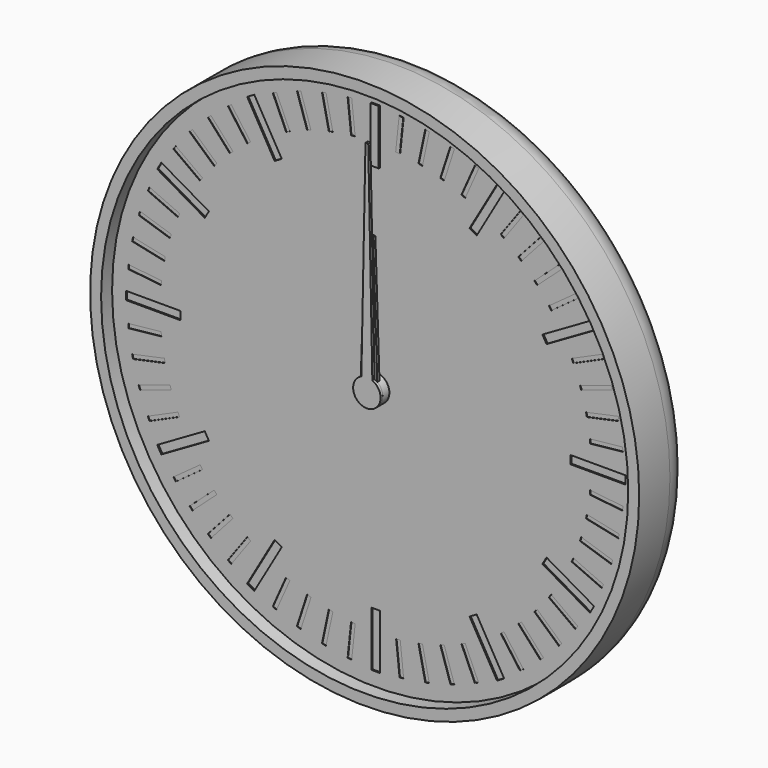
from build123d import *

# Parameters (mm, degrees)
F0_R      = 100
F1_DEPTH  = 24
F2_R      = 10
F3_T      = -4
F4_R      = 5
F4_R_2    = 3
F5_DEPTH  = 2
F6_DEPTH  = 19
F7_DEPTH  = 8
F9_DEPTH  = 4
F11_DEPTH = 4
F12_R     = 5
F12_R_2   = 3
F13_DEPTH = 2
F14_R     = 3
F15_DEPTH = 4
F17_DEPTH = 4
F18_R     = 3
F19_DEPTH = 2
F20_R     = 98
F20_R_2   = 5
F21_DEPTH = 1
F23_R     = 5
F23_R_2   = 3
F24_DEPTH = 2
F25_W     = 3
F25_H     = 20
F25_W_2   = 20
F25_H_2   = 3
F26_DEPTH = 0.5
F27_W     = 1.5
F27_H     = 12
F27_W_2   = 12
F27_H_2   = 1.5
F28_DEPTH = 0.2
F29_DEPTH = 1
F30_DEPTH = 0.4
F31_R     = 5
F31_R_2   = 3
F32_DEPTH = 5
F33_R     = 3
F34_DEPTH = 1
F36_DEPTH = 1


with BuildPart() as f1:
    # F0 (on Front) → F1 (new body)
    with BuildSketch(Plane.XZ):
        Circle(F0_R)
    extrude(amount=F1_DEPTH)

    # F2
    f2_edges = [f1.edges().sort_by_distance(p)[0] for p in [
        (-100, 0, 0),
    ]]
    fillet(f2_edges, radius=F2_R)

    # F3
    f3_openings = [f1.faces().sort_by_distance(p)[0] for p in [
        (0, -24, 0),
    ]]
    offset(amount=F3_T, openings=f3_openings)

    # F4 (on face) → F5 (join)
    with BuildSketch(Plane.XZ.offset(4)):
        Circle(F4_R)
        Circle(F4_R_2, mode=Mode.SUBTRACT)
        with Locations((40, 0)):
            Circle(F4_R)
        with Locations((40, 0)):
            Circle(F4_R_2, mode=Mode.SUBTRACT)
    extrude(amount=F5_DEPTH)


with BuildPart() as f6:
    # F6 (new): a face of the model
    f6_faces = [f1.part.faces().sort_by_distance(p)[0] for p in [
        (0, -4, 0),
    ]]
    extrude(f6_faces, amount=F6_DEPTH)

    # F8 (on face) → F9 (join)
    with BuildSketch(Plane.XZ.offset(6)):
        with BuildLine():
            ThreePointArc((9.2729637667, -1.3794085621), (9.3494561423, -0.6915886375), (9.375, 0))
            ThreePointArc((9.375, 0), (9.3494561423, 0.6915886375), (9.2729637667, 1.3794085621))
            ThreePointArc((9.2729637667, 1.3794085621), (8.9161548403, 2.8970343223), (8.3127812852, 4.3345463782))
            ThreePointArc((8.3127812852, 4.3345463782), (7.5845343223, 5.5104867402), (6.6911892658, 6.566476316))
            ThreePointArc((6.6911892658, 6.566476316), (5.5104867402, 7.5845343223), (4.1773988938, 8.3928519278))
            ThreePointArc((4.1773988938, 8.3928519278), (2.8970343223, 8.9161548403), (1.5536078905, 9.2453733036))
            ThreePointArc((1.5536078905, 9.2453733036), (0, 9.375), (-1.5536078905, 9.2453733036))
            ThreePointArc((-1.5536078905, 9.2453733036), (-2.8970343223, 8.9161548403), (-4.1773988938, 8.3928519278))
            ThreePointArc((-4.1773988938, 8.3928519278), (-5.5104867402, 7.5845343223), (-6.6911892658, 6.566476316))
            ThreePointArc((-6.6911892658, 6.566476316), (-7.5845343223, 5.5104867402), (-8.3127812852, 4.3345463782))
            ThreePointArc((-8.3127812852, 4.3345463782), (-8.9161548403, 2.8970343223), (-9.2729637667, 1.3794085621))
            ThreePointArc((-9.2729637667, 1.3794085621), (-9.375, 0), (-9.2729637667, -1.3794085621))
            ThreePointArc((-9.2729637667, -1.3794085621), (-8.9161548403, -2.8970343223), (-8.3127812852, -4.3345463782))
            ThreePointArc((-8.3127812852, -4.3345463782), (-7.5845343223, -5.5104867402), (-6.6911892658, -6.566476316))
            ThreePointArc((-6.6911892658, -6.566476316), (-5.5104867402, -7.5845343223), (-4.1773988938, -8.3928519278))
            ThreePointArc((-4.1773988938, -8.3928519278), (-2.8970343223, -8.9161548403), (-1.5536078905, -9.2453733036))
            ThreePointArc((-1.5536078905, -9.2453733036), (0, -9.375), (1.5536078905, -9.2453733036))
            ThreePointArc((1.5536078905, -9.2453733036), (2.8970343223, -8.9161548403), (4.1773988938, -8.3928519278))
            ThreePointArc((4.1773988938, -8.3928519278), (5.5104867402, -7.5845343223), (6.6911892658, -6.566476316))
            ThreePointArc((6.6911892658, -6.566476316), (7.5845343223, -5.5104867402), (8.3127812852, -4.3345463782))
            ThreePointArc((8.3127812852, -4.3345463782), (8.9161548403, -2.8970343223), (9.2729637667, -1.3794085621))
        make_face()
        with BuildLine():
            ThreePointArc((8.3127812852, 4.3345463782), (8.9161548403, 2.8970343223), (9.2729637667, 1.3794085621))
            Line((9.2729637667, 1.3794085621), (11.1823199426, 2.3946312492))
            Line((11.1823199426, 2.3946312492), (10.8182678729, 3.515068311))
            Line((10.8182678729, 3.515068311), (10.4542158031, 4.6355053728))
            Line((10.4542158031, 4.6355053728), (8.3127812852, 4.3345463782))
        make_face()
        with BuildLine():
            Line((11.1823199426, -2.3946312492), (9.2729637667, -1.3794085621))
            ThreePointArc((9.2729637667, -1.3794085621), (8.9161548403, -2.8970343223), (8.3127812852, -4.3345463782))
            Line((8.3127812852, -4.3345463782), (10.4542158031, -4.6355053728))
            Line((10.4542158031, -4.6355053728), (10.8182678729, -3.515068311))
            Line((10.8182678729, -3.515068311), (11.1823199426, -2.3946312492))
        make_face()
        with BuildLine():
            ThreePointArc((4.1773988938, 8.3928519278), (5.5104867402, 7.5845343223), (6.6911892658, 6.566476316))
            Line((6.6911892658, 6.566476316), (7.6391579371, 8.5101001246))
            Line((7.6391579371, 8.5101001246), (6.6860572448, 9.202568311))
            Line((6.6860572448, 9.202568311), (5.7329565525, 9.8950364974))
            Line((5.7329565525, 9.8950364974), (4.1773988938, 8.3928519278))
        make_face()
        with BuildLine():
            Line((7.6391579371, -8.5101001246), (6.6911892658, -6.566476316))
            ThreePointArc((6.6911892658, -6.566476316), (5.5104867402, -7.5845343223), (4.1773988938, -8.3928519278))
            Line((4.1773988938, -8.3928519278), (5.7329565525, -9.8950364974))
            Line((5.7329565525, -9.8950364974), (6.6860572448, -9.202568311))
            Line((6.6860572448, -9.202568311), (7.6391579371, -8.5101001246))
        make_face()
        with BuildLine():
            ThreePointArc((-1.5536078905, 9.2453733036), (0, 9.375), (1.5536078905, 9.2453733036))
            Line((1.5536078905, 9.2453733036), (1.1780972451, 11.375))
            Line((1.1780972451, 11.375), (0, 11.375))
            Line((0, 11.375), (-1.1780972451, 11.375))
            Line((-1.1780972451, 11.375), (-1.5536078905, 9.2453733036))
        make_face()
        with BuildLine():
            Line((1.1780972451, -11.375), (1.5536078905, -9.2453733036))
            ThreePointArc((1.5536078905, -9.2453733036), (0, -9.375), (-1.5536078905, -9.2453733036))
            Line((-1.5536078905, -9.2453733036), (-1.1780972451, -11.375))
            Line((-1.1780972451, -11.375), (0, -11.375))
            Line((0, -11.375), (1.1780972451, -11.375))
        make_face()
        with BuildLine():
            ThreePointArc((-6.6911892658, 6.566476316), (-5.5104867402, 7.5845343223), (-4.1773988938, 8.3928519278))
            Line((-4.1773988938, 8.3928519278), (-5.7329565525, 9.8950364974))
            Line((-5.7329565525, 9.8950364974), (-6.6860572448, 9.202568311))
            Line((-6.6860572448, 9.202568311), (-7.6391579371, 8.5101001246))
            Line((-7.6391579371, 8.5101001246), (-6.6911892658, 6.566476316))
        make_face()
        with BuildLine():
            Line((-5.7329565525, -9.8950364974), (-4.1773988938, -8.3928519278))
            ThreePointArc((-4.1773988938, -8.3928519278), (-5.5104867402, -7.5845343223), (-6.6911892658, -6.566476316))
            Line((-6.6911892658, -6.566476316), (-7.6391579371, -8.5101001246))
            Line((-7.6391579371, -8.5101001246), (-6.6860572448, -9.202568311))
            Line((-6.6860572448, -9.202568311), (-5.7329565525, -9.8950364974))
        make_face()
        with BuildLine():
            ThreePointArc((-9.2729637667, 1.3794085621), (-8.9161548403, 2.8970343223), (-8.3127812852, 4.3345463782))
            Line((-8.3127812852, 4.3345463782), (-10.4542158031, 4.6355053728))
            Line((-10.4542158031, 4.6355053728), (-10.8182678729, 3.515068311))
            Line((-10.8182678729, 3.515068311), (-11.1823199426, 2.3946312492))
            Line((-11.1823199426, 2.3946312492), (-9.2729637667, 1.3794085621))
        make_face()
        with BuildLine():
            Line((-10.4542158031, -4.6355053728), (-8.3127812852, -4.3345463782))
            ThreePointArc((-8.3127812852, -4.3345463782), (-8.9161548403, -2.8970343223), (-9.2729637667, -1.3794085621))
            Line((-9.2729637667, -1.3794085621), (-11.1823199426, -2.3946312492))
            Line((-11.1823199426, -2.3946312492), (-10.8182678729, -3.515068311))
            Line((-10.8182678729, -3.515068311), (-10.4542158031, -4.6355053728))
        make_face()
    extrude(amount=F9_DEPTH)

    # F35 (on face) → F36 (join)
    with BuildSketch(Plane.XZ.offset(23)):
        with BuildLine():
            ThreePointArc((-2, 4.582575695), (-2.7386127875, -4.1833001327), (5, 0))
            ThreePointArc((5, 0), (4.1833001327, 2.7386127875), (2, 4.582575695))
            ThreePointArc((2, 4.582575695), (0, 5), (-2, 4.582575695))
        make_face()
        with BuildLine():
            ThreePointArc((-2, 4.582575695), (0, 5), (2, 4.582575695))
            Line((2, 4.582575695), (0.5, 80))
            Line((0.5, 80), (0, 80))
            Line((0, 80), (-0.5, 80))
            Line((-0.5, 80), (-2, 4.582575695))
        make_face()
    extrude(amount=-F36_DEPTH)


with BuildPart() as f7:
    # F7 (new): a face of the model
    f7_faces = [f1.part.faces().sort_by_distance(p)[0] for p in [
        (40, -4, 0),
    ]]
    extrude(f7_faces, amount=F7_DEPTH)

    # F10 (on face) → F11 (join)
    with BuildSketch(Plane.XZ.offset(6)):
        with BuildLine():
            ThreePointArc((68.0829066802, -1.5381733945), (68.1144747006, -0.7693746225), (68.125, 0))
            ThreePointArc((68.125, 0), (68.1144747006, 0.7693746225), (68.0829066802, 1.5381733945))
            ThreePointArc((68.0829066802, 1.5381733945), (67.9709283072, 2.9398630294), (67.7890320221, 4.3342039956))
            ThreePointArc((67.7890320221, 4.3342039956), (67.5104012706, 5.8475163042), (67.1494235596, 7.3433252263))
            ThreePointArc((67.1494235596, 7.3433252263), (66.7484645208, 8.6911029668), (66.280643318, 10.0171558733))
            ThreePointArc((66.280643318, 10.0171558733), (65.6934659962, 11.4394680865), (65.0293803521, 12.8275385085))
            ThreePointArc((65.0293803521, 12.8275385085), (64.3569644814, 14.0625), (63.6236643925, 15.2623099717))
            ThreePointArc((63.6236643925, 15.2623099717), (62.7536029668, 16.5314602207), (61.815433119, 17.7511268046))
            ThreePointArc((61.815433119, 17.7511268046), (60.9009482166, 18.8192983038), (59.934217974, 19.8404278876))
            ThreePointArc((59.934217974, 19.8404278876), (58.8192983038, 20.9009482166), (57.6480467764, 21.8989056799))
            ThreePointArc((57.6480467764, 21.8989056799), (56.5314602207, 22.7536029668), (55.3735505752, 23.5514238999))
            ThreePointArc((55.3735505752, 23.5514238999), (54.0625, 24.3569644814), (52.709356105, 25.0895972944))
            ThreePointArc((52.709356105, 25.0895972944), (51.4394680865, 25.6934659962), (50.1409852457, 26.2331096755))
            ThreePointArc((50.1409852457, 26.2331096755), (48.6911029668, 26.7484645208), (47.2152055856, 27.1837531139))
            ThreePointArc((47.2152055856, 27.1837531139), (45.8475163042, 27.5104012706), (44.4652101991, 27.7682826779))
            ThreePointArc((44.4652101991, 27.7682826779), (42.9398630294, 27.9709283072), (41.4057159597, 28.0898484802))
            ThreePointArc((41.4057159597, 28.0898484802), (40, 28.125), (38.5942840403, 28.0898484802))
            ThreePointArc((38.5942840403, 28.0898484802), (37.0601369706, 27.9709283072), (35.5347898009, 27.7682826779))
            ThreePointArc((35.5347898009, 27.7682826779), (34.1524836958, 27.5104012706), (32.7847944144, 27.1837531139))
            ThreePointArc((32.7847944144, 27.1837531139), (31.3088970332, 26.7484645208), (29.8590147543, 26.2331096755))
            ThreePointArc((29.8590147543, 26.2331096755), (28.5605319135, 25.6934659962), (27.290643895, 25.0895972944))
            ThreePointArc((27.290643895, 25.0895972944), (25.9375, 24.3569644814), (24.6264494248, 23.5514238999))
            ThreePointArc((24.6264494248, 23.5514238999), (23.4685397793, 22.7536029668), (22.3519532236, 21.8989056799))
            ThreePointArc((22.3519532236, 21.8989056799), (21.1807016962, 20.9009482166), (20.065782026, 19.8404278876))
            ThreePointArc((20.065782026, 19.8404278876), (19.0990517834, 18.8192983038), (18.184566881, 17.7511268046))
            ThreePointArc((18.184566881, 17.7511268046), (17.2463970332, 16.5314602207), (16.3763356075, 15.2623099717))
            ThreePointArc((16.3763356075, 15.2623099717), (15.6430355186, 14.0625), (14.9706196479, 12.8275385085))
            ThreePointArc((14.9706196479, 12.8275385085), (14.3065340038, 11.4394680865), (13.719356682, 10.0171558733))
            ThreePointArc((13.719356682, 10.0171558733), (13.2515354792, 8.6911029668), (12.8505764404, 7.3433252263))
            ThreePointArc((12.8505764404, 7.3433252263), (12.4895987294, 5.8475163042), (12.2109679779, 4.3342039956))
            ThreePointArc((12.2109679779, 4.3342039956), (12.0290716928, 2.9398630294), (11.9170933198, 1.5381733945))
            ThreePointArc((11.9170933198, 1.5381733945), (11.875, 0), (11.9170933198, -1.5381733945))
            ThreePointArc((11.9170933198, -1.5381733945), (12.0290716928, -2.9398630294), (12.2109679779, -4.3342039956))
            ThreePointArc((12.2109679779, -4.3342039956), (12.4895987294, -5.8475163042), (12.8505764404, -7.3433252263))
            ThreePointArc((12.8505764404, -7.3433252263), (13.2515354792, -8.6911029668), (13.719356682, -10.0171558733))
            ThreePointArc((13.719356682, -10.0171558733), (14.3065340038, -11.4394680865), (14.9706196479, -12.8275385085))
            ThreePointArc((14.9706196479, -12.8275385085), (15.6430355186, -14.0625), (16.3763356075, -15.2623099717))
            ThreePointArc((16.3763356075, -15.2623099717), (17.2463970332, -16.5314602207), (18.184566881, -17.7511268046))
            ThreePointArc((18.184566881, -17.7511268046), (19.0990517834, -18.8192983038), (20.065782026, -19.8404278876))
            ThreePointArc((20.065782026, -19.8404278876), (21.1807016962, -20.9009482166), (22.3519532236, -21.8989056799))
            ThreePointArc((22.3519532236, -21.8989056799), (23.4685397793, -22.7536029668), (24.6264494248, -23.5514238999))
            ThreePointArc((24.6264494248, -23.5514238999), (25.9375, -24.3569644814), (27.290643895, -25.0895972944))
            ThreePointArc((27.290643895, -25.0895972944), (28.5605319135, -25.6934659962), (29.8590147543, -26.2331096755))
            ThreePointArc((29.8590147543, -26.2331096755), (31.3088970332, -26.7484645208), (32.7847944144, -27.1837531139))
            ThreePointArc((32.7847944144, -27.1837531139), (34.1524836958, -27.5104012706), (35.5347898009, -27.7682826779))
            ThreePointArc((35.5347898009, -27.7682826779), (37.0601369706, -27.9709283072), (38.5942840403, -28.0898484802))
            ThreePointArc((38.5942840403, -28.0898484802), (40, -28.125), (41.4057159597, -28.0898484802))
            ThreePointArc((41.4057159597, -28.0898484802), (42.9398630294, -27.9709283072), (44.4652101991, -27.7682826779))
            ThreePointArc((44.4652101991, -27.7682826779), (45.8475163042, -27.5104012706), (47.2152055856, -27.1837531139))
            ThreePointArc((47.2152055856, -27.1837531139), (48.6911029668, -26.7484645208), (50.1409852457, -26.2331096755))
            ThreePointArc((50.1409852457, -26.2331096755), (51.4394680865, -25.6934659962), (52.709356105, -25.0895972944))
            ThreePointArc((52.709356105, -25.0895972944), (54.0625, -24.3569644814), (55.3735505752, -23.5514238999))
            ThreePointArc((55.3735505752, -23.5514238999), (56.5314602207, -22.7536029668), (57.6480467764, -21.8989056799))
            ThreePointArc((57.6480467764, -21.8989056799), (58.8192983038, -20.9009482166), (59.934217974, -19.8404278876))
            ThreePointArc((59.934217974, -19.8404278876), (60.9009482166, -18.8192983038), (61.815433119, -17.7511268046))
            ThreePointArc((61.815433119, -17.7511268046), (62.7536029668, -16.5314602207), (63.6236643925, -15.2623099717))
            ThreePointArc((63.6236643925, -15.2623099717), (64.3569644814, -14.0625), (65.0293803521, -12.8275385085))
            ThreePointArc((65.0293803521, -12.8275385085), (65.6934659962, -11.4394680865), (66.280643318, -10.0171558733))
            ThreePointArc((66.280643318, -10.0171558733), (66.7484645208, -8.6911029668), (67.1494235596, -7.3433252263))
            ThreePointArc((67.1494235596, -7.3433252263), (67.5104012706, -5.8475163042), (67.7890320221, -4.3342039956))
            ThreePointArc((67.7890320221, -4.3342039956), (67.9709283072, -2.9398630294), (68.0829066802, -1.5381733945))
        make_face()
        with BuildLine():
            ThreePointArc((68.0829066802, 1.5381733945), (68.1144747006, 0.7693746225), (68.125, 0))
            ThreePointArc((68.125, 0), (68.1144747006, -0.7693746225), (68.0829066802, -1.5381733945))
            Line((68.0829066802, -1.5381733945), (70.125, -1.1780972451))
            Line((70.125, -1.1780972451), (70.125, 0))
            Line((70.125, 0), (70.125, 1.1780972451))
            Line((70.125, 1.1780972451), (68.0829066802, 1.5381733945))
        make_face()
        with BuildLine():
            ThreePointArc((67.1494235596, 7.3433252263), (67.5104012706, 5.8475163042), (67.7890320221, 4.3342039956))
            Line((67.7890320221, 4.3342039956), (69.7116366623, 5.1109866922))
            Line((69.7116366623, 5.1109866922), (69.4666964721, 6.2633396859))
            Line((69.4666964721, 6.2633396859), (69.2217562819, 7.4156926796))
            Line((69.2217562819, 7.4156926796), (67.1494235596, 7.3433252263))
        make_face()
        with BuildLine():
            Line((69.7116366623, -5.1109866922), (67.7890320221, -4.3342039956))
            ThreePointArc((67.7890320221, -4.3342039956), (67.5104012706, -5.8475163042), (67.1494235596, -7.3433252263))
            Line((67.1494235596, -7.3433252263), (69.2217562819, -7.4156926796))
            Line((69.2217562819, -7.4156926796), (69.4666964721, -6.2633396859))
            Line((69.4666964721, -6.2633396859), (69.7116366623, -5.1109866922))
        make_face()
        with BuildLine():
            ThreePointArc((65.0293803521, 12.8275385085), (65.6934659962, 11.4394680865), (66.280643318, 10.0171558733))
            Line((66.280643318, 10.0171558733), (67.9997322302, 11.1766959857))
            Line((67.9997322302, 11.1766959857), (67.5205569115, 12.2529413727))
            Line((67.5205569115, 12.2529413727), (67.0413815928, 13.3291867596))
            Line((67.0413815928, 13.3291867596), (65.0293803521, 12.8275385085))
        make_face()
        with BuildLine():
            Line((67.9997322302, -11.1766959857), (66.280643318, -10.0171558733))
            ThreePointArc((66.280643318, -10.0171558733), (65.6934659962, -11.4394680865), (65.0293803521, -12.8275385085))
            Line((65.0293803521, -12.8275385085), (67.0413815928, -13.3291867596))
            Line((67.0413815928, -13.3291867596), (67.5205569115, -12.2529413727))
            Line((67.5205569115, -12.2529413727), (67.9997322302, -11.1766959857))
        make_face()
        with BuildLine():
            ThreePointArc((61.815433119, 17.7511268046), (62.7536029668, 16.5314602207), (63.6236643925, 15.2623099717))
            Line((63.6236643925, 15.2623099717), (65.064105142, 16.753930033))
            Line((65.064105142, 16.753930033), (64.3716369555, 17.7070307253))
            Line((64.3716369555, 17.7070307253), (63.6791687691, 18.6601314176))
            Line((63.6791687691, 18.6601314176), (61.815433119, 17.7511268046))
        make_face()
        with BuildLine():
            Line((65.064105142, -16.753930033), (63.6236643925, -15.2623099717))
            ThreePointArc((63.6236643925, -15.2623099717), (62.7536029668, -16.5314602207), (61.815433119, -17.7511268046))
            Line((61.815433119, -17.7511268046), (63.6791687691, -18.6601314176))
            Line((63.6791687691, -18.6601314176), (64.3716369555, -17.7070307253))
            Line((64.3716369555, -17.7070307253), (65.064105142, -16.753930033))
        make_face()
        with BuildLine():
            ThreePointArc((57.6480467764, 21.8989056799), (58.8192983038, 20.9009482166), (59.934217974, 19.8404278876))
            Line((59.934217974, 19.8404278876), (61.0330563882, 21.5989369435))
            Line((61.0330563882, 21.5989369435), (60.1575595166, 22.3872378675))
            Line((60.1575595166, 22.3872378675), (59.282062645, 23.1755387915))
            Line((59.282062645, 23.1755387915), (57.6480467764, 21.8989056799))
        make_face()
        with BuildLine():
            Line((61.0330563882, -21.5989369435), (59.934217974, -19.8404278876))
            ThreePointArc((59.934217974, -19.8404278876), (58.8192983038, -20.9009482166), (57.6480467764, -21.8989056799))
            Line((57.6480467764, -21.8989056799), (59.282062645, -23.1755387915))
            Line((59.282062645, -23.1755387915), (60.1575595166, -22.3872378675))
            Line((60.1575595166, -22.3872378675), (61.0330563882, -21.5989369435))
        make_face()
        with BuildLine():
            ThreePointArc((52.709356105, 25.0895972944), (54.0625, 24.3569644814), (55.3735505752, 23.5514238999))
            Line((55.3735505752, 23.5514238999), (56.0827621424, 25.4999666665))
            Line((56.0827621424, 25.4999666665), (55.0625, 26.089015289))
            Line((55.0625, 26.089015289), (54.0422378576, 26.6780639116))
            Line((54.0422378576, 26.6780639116), (52.709356105, 25.0895972944))
        make_face()
        with BuildLine():
            Line((56.0827621424, -25.4999666665), (55.3735505752, -23.5514238999))
            ThreePointArc((55.3735505752, -23.5514238999), (54.0625, -24.3569644814), (52.709356105, -25.0895972944))
            Line((52.709356105, -25.0895972944), (54.0422378576, -26.6780639116))
            Line((54.0422378576, -26.6780639116), (55.0625, -26.089015289))
            Line((55.0625, -26.089015289), (56.0827621424, -25.4999666665))
        make_face()
        with BuildLine():
            ThreePointArc((47.2152055856, 27.1837531139), (48.6911029668, 26.7484645208), (50.1409852457, 26.2331096755))
            Line((50.1409852457, 26.2331096755), (50.4295740173, 28.2865254836))
            Line((50.4295740173, 28.2865254836), (49.3091369555, 28.6505775534))
            Line((49.3091369555, 28.6505775534), (48.1886998938, 29.0146296232))
            Line((48.1886998938, 29.0146296232), (47.2152055856, 27.1837531139))
        make_face()
        with BuildLine():
            Line((50.4295740173, -28.2865254836), (50.1409852457, -26.2331096755))
            ThreePointArc((50.1409852457, -26.2331096755), (48.6911029668, -26.7484645208), (47.2152055856, -27.1837531139))
            Line((47.2152055856, -27.1837531139), (48.1886998938, -29.0146296232))
            Line((48.1886998938, -29.0146296232), (49.3091369555, -28.6505775534))
            Line((49.3091369555, -28.6505775534), (50.4295740173, -28.2865254836))
        make_face()
        with BuildLine():
            ThreePointArc((41.4057159597, 28.0898484802), (42.9398630294, 27.9709283072), (44.4652101991, 27.7682826779))
            Line((44.4652101991, 27.7682826779), (44.3205634611, 29.8368274034))
            Line((44.3205634611, 29.8368274034), (43.1489199559, 29.959972098))
            Line((43.1489199559, 29.959972098), (41.9772764508, 30.0831167926))
            Line((41.9772764508, 30.0831167926), (41.4057159597, 28.0898484802))
        make_face()
        with BuildLine():
            Line((44.3205634611, -29.8368274034), (44.4652101991, -27.7682826779))
            ThreePointArc((44.4652101991, -27.7682826779), (42.9398630294, -27.9709283072), (41.4057159597, -28.0898484802))
            Line((41.4057159597, -28.0898484802), (41.9772764508, -30.0831167926))
            Line((41.9772764508, -30.0831167926), (43.1489199559, -29.959972098))
            Line((43.1489199559, -29.959972098), (44.3205634611, -29.8368274034))
        make_face()
        with BuildLine():
            ThreePointArc((35.5347898009, 27.7682826779), (37.0601369706, 27.9709283072), (38.5942840403, 28.0898484802))
            Line((38.5942840403, 28.0898484802), (38.0227235492, 30.0831167926))
            Line((38.0227235492, 30.0831167926), (36.8510800441, 29.959972098))
            Line((36.8510800441, 29.959972098), (35.6794365389, 29.8368274034))
            Line((35.6794365389, 29.8368274034), (35.5347898009, 27.7682826779))
        make_face()
        with BuildLine():
            Line((38.0227235492, -30.0831167926), (38.5942840403, -28.0898484802))
            ThreePointArc((38.5942840403, -28.0898484802), (37.0601369706, -27.9709283072), (35.5347898009, -27.7682826779))
            Line((35.5347898009, -27.7682826779), (35.6794365389, -29.8368274034))
            Line((35.6794365389, -29.8368274034), (36.8510800441, -29.959972098))
            Line((36.8510800441, -29.959972098), (38.0227235492, -30.0831167926))
        make_face()
        with BuildLine():
            ThreePointArc((29.8590147543, 26.2331096755), (31.3088970332, 26.7484645208), (32.7847944144, 27.1837531139))
            Line((32.7847944144, 27.1837531139), (31.8113001062, 29.0146296232))
            Line((31.8113001062, 29.0146296232), (30.6908630445, 28.6505775534))
            Line((30.6908630445, 28.6505775534), (29.5704259827, 28.2865254836))
            Line((29.5704259827, 28.2865254836), (29.8590147543, 26.2331096755))
        make_face()
        with BuildLine():
            Line((31.8113001062, -29.0146296232), (32.7847944144, -27.1837531139))
            ThreePointArc((32.7847944144, -27.1837531139), (31.3088970332, -26.7484645208), (29.8590147543, -26.2331096755))
            Line((29.8590147543, -26.2331096755), (29.5704259827, -28.2865254836))
            Line((29.5704259827, -28.2865254836), (30.6908630445, -28.6505775534))
            Line((30.6908630445, -28.6505775534), (31.8113001062, -29.0146296232))
        make_face()
        with BuildLine():
            ThreePointArc((24.6264494248, 23.5514238999), (25.9375, 24.3569644814), (27.290643895, 25.0895972944))
            Line((27.290643895, 25.0895972944), (25.9577621424, 26.6780639116))
            Line((25.9577621424, 26.6780639116), (24.9375, 26.089015289))
            Line((24.9375, 26.089015289), (23.9172378576, 25.4999666665))
            Line((23.9172378576, 25.4999666665), (24.6264494248, 23.5514238999))
        make_face()
        with BuildLine():
            Line((25.9577621424, -26.6780639116), (27.290643895, -25.0895972944))
            ThreePointArc((27.290643895, -25.0895972944), (25.9375, -24.3569644814), (24.6264494248, -23.5514238999))
            Line((24.6264494248, -23.5514238999), (23.9172378576, -25.4999666665))
            Line((23.9172378576, -25.4999666665), (24.9375, -26.089015289))
            Line((24.9375, -26.089015289), (25.9577621424, -26.6780639116))
        make_face()
        with BuildLine():
            ThreePointArc((20.065782026, 19.8404278876), (21.1807016962, 20.9009482166), (22.3519532236, 21.8989056799))
            Line((22.3519532236, 21.8989056799), (20.717937355, 23.1755387915))
            Line((20.717937355, 23.1755387915), (19.8424404834, 22.3872378675))
            Line((19.8424404834, 22.3872378675), (18.9669436118, 21.5989369435))
            Line((18.9669436118, 21.5989369435), (20.065782026, 19.8404278876))
        make_face()
        with BuildLine():
            Line((20.717937355, -23.1755387915), (22.3519532236, -21.8989056799))
            ThreePointArc((22.3519532236, -21.8989056799), (21.1807016962, -20.9009482166), (20.065782026, -19.8404278876))
            Line((20.065782026, -19.8404278876), (18.9669436118, -21.5989369435))
            Line((18.9669436118, -21.5989369435), (19.8424404834, -22.3872378675))
            Line((19.8424404834, -22.3872378675), (20.717937355, -23.1755387915))
        make_face()
        with BuildLine():
            ThreePointArc((16.3763356075, 15.2623099717), (17.2463970332, 16.5314602207), (18.184566881, 17.7511268046))
            Line((18.184566881, 17.7511268046), (16.3208312309, 18.6601314176))
            Line((16.3208312309, 18.6601314176), (15.6283630445, 17.7070307253))
            Line((15.6283630445, 17.7070307253), (14.935894858, 16.753930033))
            Line((14.935894858, 16.753930033), (16.3763356075, 15.2623099717))
        make_face()
        with BuildLine():
            Line((16.3208312309, -18.6601314176), (18.184566881, -17.7511268046))
            ThreePointArc((18.184566881, -17.7511268046), (17.2463970332, -16.5314602207), (16.3763356075, -15.2623099717))
            Line((16.3763356075, -15.2623099717), (14.935894858, -16.753930033))
            Line((14.935894858, -16.753930033), (15.6283630445, -17.7070307253))
            Line((15.6283630445, -17.7070307253), (16.3208312309, -18.6601314176))
        make_face()
        with BuildLine():
            ThreePointArc((13.719356682, 10.0171558733), (14.3065340038, 11.4394680865), (14.9706196479, 12.8275385085))
            Line((14.9706196479, 12.8275385085), (12.9586184072, 13.3291867596))
            Line((12.9586184072, 13.3291867596), (12.4794430885, 12.2529413727))
            Line((12.4794430885, 12.2529413727), (12.0002677698, 11.1766959857))
            Line((12.0002677698, 11.1766959857), (13.719356682, 10.0171558733))
        make_face()
        with BuildLine():
            Line((12.9586184072, -13.3291867596), (14.9706196479, -12.8275385085))
            ThreePointArc((14.9706196479, -12.8275385085), (14.3065340038, -11.4394680865), (13.719356682, -10.0171558733))
            Line((13.719356682, -10.0171558733), (12.0002677698, -11.1766959857))
            Line((12.0002677698, -11.1766959857), (12.4794430885, -12.2529413727))
            Line((12.4794430885, -12.2529413727), (12.9586184072, -13.3291867596))
        make_face()
        with BuildLine():
            ThreePointArc((12.2109679779, 4.3342039956), (12.4895987294, 5.8475163042), (12.8505764404, 7.3433252263))
            Line((12.8505764404, 7.3433252263), (10.7782437181, 7.4156926796))
            Line((10.7782437181, 7.4156926796), (10.5333035279, 6.2633396859))
            Line((10.5333035279, 6.2633396859), (10.2883633377, 5.1109866922))
            Line((10.2883633377, 5.1109866922), (12.2109679779, 4.3342039956))
        make_face()
        with BuildLine():
            Line((10.7782437181, -7.4156926796), (12.8505764404, -7.3433252263))
            ThreePointArc((12.8505764404, -7.3433252263), (12.4895987294, -5.8475163042), (12.2109679779, -4.3342039956))
            Line((12.2109679779, -4.3342039956), (10.2883633377, -5.1109866922))
            Line((10.2883633377, -5.1109866922), (10.5333035279, -6.2633396859))
            Line((10.5333035279, -6.2633396859), (10.7782437181, -7.4156926796))
        make_face()
        with BuildLine():
            ThreePointArc((11.9170933198, -1.5381733945), (11.875, 0), (11.9170933198, 1.5381733945))
            Line((11.9170933198, 1.5381733945), (9.875, 1.1780972451))
            Line((9.875, 1.1780972451), (9.875, 0))
            Line((9.875, 0), (9.875, -1.1780972451))
            Line((9.875, -1.1780972451), (11.9170933198, -1.5381733945))
        make_face()
    extrude(amount=F11_DEPTH)

    # F16 (on face) → F17 (join)
    with BuildSketch(Plane.XZ.offset(12)):
        with BuildLine():
            ThreePointArc((47.4288750323, -1.0304444454), (47.4821976298, -0.5164480894), (47.5, 0))
            ThreePointArc((47.5, 0), (47.4821976298, 0.5164480894), (47.4288750323, 1.0304444454))
            ThreePointArc((47.4288750323, 1.0304444454), (47.1329238722, 2.3176274578), (46.6157661985, 3.532936117))
            ThreePointArc((46.6157661985, 3.532936117), (46.0676274578, 4.4083893922), (45.4044061018, 5.2002302532))
            ThreePointArc((45.4044061018, 5.2002302532), (44.4083893922, 6.0676274578), (43.2756595386, 6.7468551628))
            ThreePointArc((43.2756595386, 6.7468551628), (42.3176274578, 7.1329238722), (41.3156377295, 7.3837048536))
            ThreePointArc((41.3156377295, 7.3837048536), (40, 7.5), (38.6843622705, 7.3837048536))
            ThreePointArc((38.6843622705, 7.3837048536), (37.6823725422, 7.1329238722), (36.7243404614, 6.7468551628))
            ThreePointArc((36.7243404614, 6.7468551628), (35.5916106078, 6.0676274578), (34.5955938982, 5.2002302532))
            ThreePointArc((34.5955938982, 5.2002302532), (33.9323725422, 4.4083893922), (33.3842338015, 3.532936117))
            ThreePointArc((33.3842338015, 3.532936117), (32.8670761278, 2.3176274578), (32.5711249677, 1.0304444454))
            ThreePointArc((32.5711249677, 1.0304444454), (32.5, 0), (32.5711249677, -1.0304444454))
            ThreePointArc((32.5711249677, -1.0304444454), (32.8670761278, -2.3176274578), (33.3842338015, -3.532936117))
            ThreePointArc((33.3842338015, -3.532936117), (33.9323725422, -4.4083893922), (34.5955938982, -5.2002302532))
            ThreePointArc((34.5955938982, -5.2002302532), (35.5916106078, -6.0676274578), (36.7243404614, -6.7468551628))
            ThreePointArc((36.7243404614, -6.7468551628), (37.6823725422, -7.1329238722), (38.6843622705, -7.3837048536))
            ThreePointArc((38.6843622705, -7.3837048536), (40, -7.5), (41.3156377295, -7.3837048536))
            ThreePointArc((41.3156377295, -7.3837048536), (42.3176274578, -7.1329238722), (43.2756595386, -6.7468551628))
            ThreePointArc((43.2756595386, -6.7468551628), (44.4083893922, -6.0676274578), (45.4044061018, -5.2002302532))
            ThreePointArc((45.4044061018, -5.2002302532), (46.0676274578, -4.4083893922), (46.6157661985, -3.532936117))
            ThreePointArc((46.6157661985, -3.532936117), (47.1329238722, -2.3176274578), (47.4288750323, -1.0304444454))
        make_face()
        with BuildLine():
            ThreePointArc((46.6157661985, 3.532936117), (47.1329238722, 2.3176274578), (47.4288750323, 1.0304444454))
            Line((47.4288750323, 1.0304444454), (49.3262785606, 2.0393117971))
            Line((49.3262785606, 2.0393117971), (48.743795249, 3.832011096))
            Line((48.743795249, 3.832011096), (46.6157661985, 3.532936117))
        make_face()
        with BuildLine():
            Line((49.3262785606, -2.0393117971), (47.4288750323, -1.0304444454))
            ThreePointArc((47.4288750323, -1.0304444454), (47.1329238722, -2.3176274578), (46.6157661985, -3.532936117))
            Line((46.6157661985, -3.532936117), (48.743795249, -3.832011096))
            Line((48.743795249, -3.832011096), (49.3262785606, -2.0393117971))
        make_face()
        with BuildLine():
            ThreePointArc((43.2756595386, 6.7468551628), (44.4083893922, 6.0676274578), (45.4044061018, 5.2002302532))
            Line((45.4044061018, 5.2002302532), (46.3464404506, 7.1316868974))
            Line((46.3464404506, 7.1316868974), (44.8214793429, 8.2396359957))
            Line((44.8214793429, 8.2396359957), (43.2756595386, 6.7468551628))
        make_face()
        with BuildLine():
            Line((46.3464404506, -7.1316868974), (45.4044061018, -5.2002302532))
            ThreePointArc((45.4044061018, -5.2002302532), (44.4083893922, -6.0676274578), (43.2756595386, -6.7468551628))
            Line((43.2756595386, -6.7468551628), (44.8214793429, -8.2396359957))
            Line((44.8214793429, -8.2396359957), (46.3464404506, -7.1316868974))
        make_face()
        with BuildLine():
            ThreePointArc((38.6843622705, 7.3837048536), (40, 7.5), (41.3156377295, 7.3837048536))
            Line((41.3156377295, 7.3837048536), (40.9424777961, 9.5))
            Line((40.9424777961, 9.5), (39.0575222039, 9.5))
            Line((39.0575222039, 9.5), (38.6843622705, 7.3837048536))
        make_face()
        with BuildLine():
            Line((40.9424777961, -9.5), (41.3156377295, -7.3837048536))
            ThreePointArc((41.3156377295, -7.3837048536), (40, -7.5), (38.6843622705, -7.3837048536))
            Line((38.6843622705, -7.3837048536), (39.0575222039, -9.5))
            Line((39.0575222039, -9.5), (40.9424777961, -9.5))
        make_face()
        with BuildLine():
            ThreePointArc((34.5955938982, 5.2002302532), (35.5916106078, 6.0676274578), (36.7243404614, 6.7468551628))
            Line((36.7243404614, 6.7468551628), (35.1785206571, 8.2396359957))
            Line((35.1785206571, 8.2396359957), (33.6535595494, 7.1316868974))
            Line((33.6535595494, 7.1316868974), (34.5955938982, 5.2002302532))
        make_face()
        with BuildLine():
            Line((35.1785206571, -8.2396359957), (36.7243404614, -6.7468551628))
            ThreePointArc((36.7243404614, -6.7468551628), (35.5916106078, -6.0676274578), (34.5955938982, -5.2002302532))
            Line((34.5955938982, -5.2002302532), (33.6535595494, -7.1316868974))
            Line((33.6535595494, -7.1316868974), (35.1785206571, -8.2396359957))
        make_face()
        with BuildLine():
            ThreePointArc((32.5711249677, 1.0304444454), (32.8670761278, 2.3176274578), (33.3842338015, 3.532936117))
            Line((33.3842338015, 3.532936117), (31.256204751, 3.832011096))
            Line((31.256204751, 3.832011096), (30.6737214394, 2.0393117971))
            Line((30.6737214394, 2.0393117971), (32.5711249677, 1.0304444454))
        make_face()
        with BuildLine():
            Line((31.256204751, -3.832011096), (33.3842338015, -3.532936117))
            ThreePointArc((33.3842338015, -3.532936117), (32.8670761278, -2.3176274578), (32.5711249677, -1.0304444454))
            Line((32.5711249677, -1.0304444454), (30.6737214394, -2.0393117971))
            Line((30.6737214394, -2.0393117971), (31.256204751, -3.832011096))
        make_face()
    extrude(amount=F17_DEPTH)

    # F18 (on face) → F19 (join)
    with BuildSketch(Plane.XZ.offset(16)):
        with Locations((40, 0)):
            Circle(F18_R)
    extrude(amount=F19_DEPTH)


with BuildPart() as f13:
    # F12 (on face) → F13 (new body)
    with BuildSketch(Plane.XZ.offset(10)):
        Circle(F12_R)
        Circle(F12_R_2, mode=Mode.SUBTRACT)
    extrude(amount=F13_DEPTH)

    # F14 (on face) → F15 (join)
    with BuildSketch(Plane.XZ.offset(12)):
        with BuildLine():
            ThreePointArc((29.9718156995, -1.3001014101), (29.9929530972, -0.6502034357), (30, 0))
            ThreePointArc((30, 0), (29.9929530972, 0.6502034357), (29.9718156995, 1.3001014101))
            ThreePointArc((29.9718156995, 1.3001014101), (29.907520012, 2.3537728718), (29.8061935814, 3.4045299509))
            ThreePointArc((29.8061935814, 3.4045299509), (29.6306502179, 4.6930339512), (29.3994322443, 5.9727199596))
            ThreePointArc((29.3994322443, 5.9727199596), (29.1710976119, 7.0033609157), (28.9066440563, 8.0253304855))
            ThreePointArc((28.9066440563, 8.0253304855), (28.5316954889, 9.2705098312), (28.1031371961, 10.4982703213))
            ThreePointArc((28.1031371961, 10.4982703213), (27.7163859753, 11.480502971), (27.2953170189, 12.448520749))
            ThreePointArc((27.2953170189, 12.448520749), (26.7301957257, 13.6197149922), (26.1148496411, 14.765318426))
            ThreePointArc((26.1148496411, 14.765318426), (25.5792049306, 15.6749569415), (25.0118886885, 16.5651871174))
            ThreePointArc((25.0118886885, 16.5651871174), (24.2705098312, 17.6335575688), (23.4835278178, 18.6687953878))
            ThreePointArc((23.4835278178, 18.6687953878), (22.812178968, 19.4834414499), (22.1125846489, 20.2739636023))
            ThreePointArc((22.1125846489, 20.2739636023), (21.2132034356, 21.2132034356), (20.2739636023, 22.1125846489))
            ThreePointArc((20.2739636023, 22.1125846489), (19.4834414499, 22.812178968), (18.6687953878, 23.4835278178))
            ThreePointArc((18.6687953878, 23.4835278178), (17.6335575688, 24.2705098312), (16.5651871174, 25.0118886885))
            ThreePointArc((16.5651871174, 25.0118886885), (15.6749569415, 25.5792049306), (14.765318426, 26.1148496411))
            ThreePointArc((14.765318426, 26.1148496411), (13.6197149922, 26.7301957257), (12.448520749, 27.2953170189))
            ThreePointArc((12.448520749, 27.2953170189), (11.480502971, 27.7163859753), (10.4982703213, 28.1031371961))
            ThreePointArc((10.4982703213, 28.1031371961), (9.2705098312, 28.5316954889), (8.0253304855, 28.9066440563))
            ThreePointArc((8.0253304855, 28.9066440563), (7.0033609157, 29.1710976119), (5.9727199596, 29.3994322443))
            ThreePointArc((5.9727199596, 29.3994322443), (4.6930339512, 29.6306502179), (3.4045299509, 29.8061935814))
            ThreePointArc((3.4045299509, 29.8061935814), (2.3537728718, 29.907520012), (1.3001014101, 29.9718156995))
            ThreePointArc((1.3001014101, 29.9718156995), (0, 30), (-1.3001014101, 29.9718156995))
            ThreePointArc((-1.3001014101, 29.9718156995), (-2.3537728718, 29.907520012), (-3.4045299509, 29.8061935814))
            ThreePointArc((-3.4045299509, 29.8061935814), (-4.6930339512, 29.6306502179), (-5.9727199596, 29.3994322443))
            ThreePointArc((-5.9727199596, 29.3994322443), (-7.0033609157, 29.1710976119), (-8.0253304855, 28.9066440563))
            ThreePointArc((-8.0253304855, 28.9066440563), (-9.2705098312, 28.5316954889), (-10.4982703213, 28.1031371961))
            ThreePointArc((-10.4982703213, 28.1031371961), (-11.480502971, 27.7163859753), (-12.448520749, 27.2953170189))
            ThreePointArc((-12.448520749, 27.2953170189), (-13.6197149922, 26.7301957257), (-14.765318426, 26.1148496411))
            ThreePointArc((-14.765318426, 26.1148496411), (-15.6749569415, 25.5792049306), (-16.5651871174, 25.0118886885))
            ThreePointArc((-16.5651871174, 25.0118886885), (-17.6335575688, 24.2705098312), (-18.6687953878, 23.4835278178))
            ThreePointArc((-18.6687953878, 23.4835278178), (-19.4834414499, 22.812178968), (-20.2739636023, 22.1125846489))
            ThreePointArc((-20.2739636023, 22.1125846489), (-21.2132034356, 21.2132034356), (-22.1125846489, 20.2739636023))
            ThreePointArc((-22.1125846489, 20.2739636023), (-22.812178968, 19.4834414499), (-23.4835278178, 18.6687953878))
            ThreePointArc((-23.4835278178, 18.6687953878), (-24.2705098312, 17.6335575688), (-25.0118886885, 16.5651871174))
            ThreePointArc((-25.0118886885, 16.5651871174), (-25.5792049306, 15.6749569415), (-26.1148496411, 14.765318426))
            ThreePointArc((-26.1148496411, 14.765318426), (-26.7301957257, 13.6197149922), (-27.2953170189, 12.448520749))
            ThreePointArc((-27.2953170189, 12.448520749), (-27.7163859753, 11.480502971), (-28.1031371961, 10.4982703213))
            ThreePointArc((-28.1031371961, 10.4982703213), (-28.5316954889, 9.2705098312), (-28.9066440563, 8.0253304855))
            ThreePointArc((-28.9066440563, 8.0253304855), (-29.1710976119, 7.0033609157), (-29.3994322443, 5.9727199596))
            ThreePointArc((-29.3994322443, 5.9727199596), (-29.6306502179, 4.6930339512), (-29.8061935814, 3.4045299509))
            ThreePointArc((-29.8061935814, 3.4045299509), (-29.907520012, 2.3537728718), (-29.9718156995, 1.3001014101))
            ThreePointArc((-29.9718156995, 1.3001014101), (-30, 0), (-29.9718156995, -1.3001014101))
            ThreePointArc((-29.9718156995, -1.3001014101), (-29.907520012, -2.3537728718), (-29.8061935814, -3.4045299509))
            ThreePointArc((-29.8061935814, -3.4045299509), (-29.6306502179, -4.6930339512), (-29.3994322443, -5.9727199596))
            ThreePointArc((-29.3994322443, -5.9727199596), (-29.1710976119, -7.0033609157), (-28.9066440563, -8.0253304855))
            ThreePointArc((-28.9066440563, -8.0253304855), (-28.5316954889, -9.2705098312), (-28.1031371961, -10.4982703213))
            ThreePointArc((-28.1031371961, -10.4982703213), (-27.7163859753, -11.480502971), (-27.2953170189, -12.448520749))
            ThreePointArc((-27.2953170189, -12.448520749), (-26.7301957257, -13.6197149922), (-26.1148496411, -14.765318426))
            ThreePointArc((-26.1148496411, -14.765318426), (-25.5792049306, -15.6749569415), (-25.0118886885, -16.5651871174))
            ThreePointArc((-25.0118886885, -16.5651871174), (-24.2705098312, -17.6335575688), (-23.4835278178, -18.6687953878))
            ThreePointArc((-23.4835278178, -18.6687953878), (-22.812178968, -19.4834414499), (-22.1125846489, -20.2739636023))
            ThreePointArc((-22.1125846489, -20.2739636023), (-21.2132034356, -21.2132034356), (-20.2739636023, -22.1125846489))
            ThreePointArc((-20.2739636023, -22.1125846489), (-19.4834414499, -22.812178968), (-18.6687953878, -23.4835278178))
            ThreePointArc((-18.6687953878, -23.4835278178), (-17.6335575688, -24.2705098312), (-16.5651871174, -25.0118886885))
            ThreePointArc((-16.5651871174, -25.0118886885), (-15.6749569415, -25.5792049306), (-14.765318426, -26.1148496411))
            ThreePointArc((-14.765318426, -26.1148496411), (-13.6197149922, -26.7301957257), (-12.448520749, -27.2953170189))
            ThreePointArc((-12.448520749, -27.2953170189), (-11.480502971, -27.7163859753), (-10.4982703213, -28.1031371961))
            ThreePointArc((-10.4982703213, -28.1031371961), (-9.2705098312, -28.5316954889), (-8.0253304855, -28.9066440563))
            ThreePointArc((-8.0253304855, -28.9066440563), (-7.0033609157, -29.1710976119), (-5.9727199596, -29.3994322443))
            ThreePointArc((-5.9727199596, -29.3994322443), (-4.6930339512, -29.6306502179), (-3.4045299509, -29.8061935814))
            ThreePointArc((-3.4045299509, -29.8061935814), (-2.3537728718, -29.907520012), (-1.3001014101, -29.9718156995))
            ThreePointArc((-1.3001014101, -29.9718156995), (0, -30), (1.3001014101, -29.9718156995))
            ThreePointArc((1.3001014101, -29.9718156995), (2.3537728718, -29.907520012), (3.4045299509, -29.8061935814))
            ThreePointArc((3.4045299509, -29.8061935814), (4.6930339512, -29.6306502179), (5.9727199596, -29.3994322443))
            ThreePointArc((5.9727199596, -29.3994322443), (7.0033609157, -29.1710976119), (8.0253304855, -28.9066440563))
            ThreePointArc((8.0253304855, -28.9066440563), (9.2705098312, -28.5316954889), (10.4982703213, -28.1031371961))
            ThreePointArc((10.4982703213, -28.1031371961), (11.480502971, -27.7163859753), (12.448520749, -27.2953170189))
            ThreePointArc((12.448520749, -27.2953170189), (13.6197149922, -26.7301957257), (14.765318426, -26.1148496411))
            ThreePointArc((14.765318426, -26.1148496411), (15.6749569415, -25.5792049306), (16.5651871174, -25.0118886885))
            ThreePointArc((16.5651871174, -25.0118886885), (17.6335575688, -24.2705098312), (18.6687953878, -23.4835278178))
            ThreePointArc((18.6687953878, -23.4835278178), (19.4834414499, -22.812178968), (20.2739636023, -22.1125846489))
            ThreePointArc((20.2739636023, -22.1125846489), (21.2132034356, -21.2132034356), (22.1125846489, -20.2739636023))
            ThreePointArc((22.1125846489, -20.2739636023), (22.812178968, -19.4834414499), (23.4835278178, -18.6687953878))
            ThreePointArc((23.4835278178, -18.6687953878), (24.2705098312, -17.6335575688), (25.0118886885, -16.5651871174))
            ThreePointArc((25.0118886885, -16.5651871174), (25.5792049306, -15.6749569415), (26.1148496411, -14.765318426))
            ThreePointArc((26.1148496411, -14.765318426), (26.7301957257, -13.6197149922), (27.2953170189, -12.448520749))
            ThreePointArc((27.2953170189, -12.448520749), (27.7163859753, -11.480502971), (28.1031371961, -10.4982703213))
            ThreePointArc((28.1031371961, -10.4982703213), (28.5316954889, -9.2705098312), (28.9066440563, -8.0253304855))
            ThreePointArc((28.9066440563, -8.0253304855), (29.1710976119, -7.0033609157), (29.3994322443, -5.9727199596))
            ThreePointArc((29.3994322443, -5.9727199596), (29.6306502179, -4.6930339512), (29.8061935814, -3.4045299509))
            ThreePointArc((29.8061935814, -3.4045299509), (29.907520012, -2.3537728718), (29.9718156995, -1.3001014101))
        make_face()
        Circle(F14_R, mode=Mode.SUBTRACT)
        with BuildLine():
            ThreePointArc((29.9718156995, 1.3001014101), (29.9929530972, 0.6502034357), (30, 0))
            ThreePointArc((30, 0), (29.9929530972, -0.6502034357), (29.9718156995, -1.3001014101))
            Line((29.9718156995, -1.3001014101), (32, -0.9424777961))
            Line((32, -0.9424777961), (32, 0))
            Line((32, 0), (32, 0.9424777961))
            Line((32, 0.9424777961), (29.9718156995, 1.3001014101))
        make_face()
        with BuildLine():
            ThreePointArc((29.3994322443, 5.9727199596), (29.6306502179, 4.6930339512), (29.8061935814, 3.4045299509))
            Line((29.8061935814, 3.4045299509), (31.7534629089, 4.0750285508))
            Line((31.7534629089, 4.0750285508), (31.606026899, 5.0059028813))
            Line((31.606026899, 5.0059028813), (31.4585908892, 5.9367772117))
            Line((31.4585908892, 5.9367772117), (29.3994322443, 5.9727199596))
        make_face()
        with BuildLine():
            Line((31.7534629089, -4.0750285508), (29.8061935814, -3.4045299509))
            ThreePointArc((29.8061935814, -3.4045299509), (29.6306502179, -4.6930339512), (29.3994322443, -5.9727199596))
            Line((29.3994322443, -5.9727199596), (31.4585908892, -5.9367772117))
            Line((31.4585908892, -5.9367772117), (31.606026899, -5.0059028813))
            Line((31.606026899, -5.0059028813), (31.7534629089, -4.0750285508))
        make_face()
        with BuildLine():
            ThreePointArc((28.1031371961, 10.4982703213), (28.5316954889, 9.2705098312), (28.9066440563, 8.0253304855))
            Line((28.9066440563, 8.0253304855), (30.7250501773, 8.9921941706))
            Line((30.7250501773, 8.9921941706), (30.4338085214, 9.88854382))
            Line((30.4338085214, 9.88854382), (30.1425668656, 10.7848934694))
            Line((30.1425668656, 10.7848934694), (28.1031371961, 10.4982703213))
        make_face()
        with BuildLine():
            Line((30.7250501773, -8.9921941706), (28.9066440563, -8.0253304855))
            ThreePointArc((28.9066440563, -8.0253304855), (28.5316954889, -9.2705098312), (28.1031371961, -10.4982703213))
            Line((28.1031371961, -10.4982703213), (30.1425668656, -10.7848934694))
            Line((30.1425668656, -10.7848934694), (30.4338085214, -9.88854382))
            Line((30.4338085214, -9.88854382), (30.7250501773, -8.9921941706))
        make_face()
        with BuildLine():
            ThreePointArc((26.1148496411, 14.765318426), (26.7301957257, 13.6197149922), (27.2953170189, 12.448520749))
            Line((27.2953170189, 12.448520749), (28.9400847397, 13.6879421265))
            Line((28.9400847397, 13.6879421265), (28.512208774, 14.5276959917))
            Line((28.512208774, 14.5276959917), (28.0843328084, 15.3674498569))
            Line((28.0843328084, 15.3674498569), (26.1148496411, 14.765318426))
        make_face()
        with BuildLine():
            Line((28.9400847397, -13.6879421265), (27.2953170189, -12.448520749))
            ThreePointArc((27.2953170189, -12.448520749), (26.7301957257, -13.6197149922), (26.1148496411, -14.765318426))
            Line((26.1148496411, -14.765318426), (28.0843328084, -15.3674498569))
            Line((28.0843328084, -15.3674498569), (28.512208774, -14.5276959917))
            Line((28.512208774, -14.5276959917), (28.9400847397, -13.6879421265))
        make_face()
        with BuildLine():
            ThreePointArc((23.4835278178, 18.6687953878), (24.2705098312, 17.6335575688), (25.0118886885, 16.5651871174))
            Line((25.0118886885, 16.5651871174), (26.4425183691, 18.0466475195))
            Line((26.4425183691, 18.0466475195), (25.88854382, 18.8091280734))
            Line((25.88854382, 18.8091280734), (25.3345692709, 19.5716086272))
            Line((25.3345692709, 19.5716086272), (23.4835278178, 18.6687953878))
        make_face()
        with BuildLine():
            Line((26.4425183691, -18.0466475195), (25.0118886885, -16.5651871174))
            ThreePointArc((25.0118886885, -16.5651871174), (24.2705098312, -17.6335575688), (23.4835278178, -18.6687953878))
            Line((23.4835278178, -18.6687953878), (25.3345692709, -19.5716086272))
            Line((25.3345692709, -19.5716086272), (25.88854382, -18.8091280734))
            Line((25.88854382, -18.8091280734), (26.4425183691, -18.0466475195))
        make_face()
        with BuildLine():
            ThreePointArc((20.2739636023, 22.1125846489), (21.2132034356, 21.2132034356), (22.1125846489, 20.2739636023))
            Line((22.1125846489, 20.2739636023), (23.2938494387, 21.9609845572))
            Line((23.2938494387, 21.9609845572), (22.627416998, 22.627416998))
            Line((22.627416998, 22.627416998), (21.9609845572, 23.2938494387))
            Line((21.9609845572, 23.2938494387), (20.2739636023, 22.1125846489))
        make_face()
        with BuildLine():
            Line((23.2938494387, -21.9609845572), (22.1125846489, -20.2739636023))
            ThreePointArc((22.1125846489, -20.2739636023), (21.2132034356, -21.2132034356), (20.2739636023, -22.1125846489))
            Line((20.2739636023, -22.1125846489), (21.9609845572, -23.2938494387))
            Line((21.9609845572, -23.2938494387), (22.627416998, -22.627416998))
            Line((22.627416998, -22.627416998), (23.2938494387, -21.9609845572))
        make_face()
        with BuildLine():
            ThreePointArc((16.5651871174, 25.0118886885), (17.6335575688, 24.2705098312), (18.6687953878, 23.4835278178))
            Line((18.6687953878, 23.4835278178), (19.5716086272, 25.3345692709))
            Line((19.5716086272, 25.3345692709), (18.8091280734, 25.88854382))
            Line((18.8091280734, 25.88854382), (18.0466475195, 26.4425183691))
            Line((18.0466475195, 26.4425183691), (16.5651871174, 25.0118886885))
        make_face()
        with BuildLine():
            Line((19.5716086272, -25.3345692709), (18.6687953878, -23.4835278178))
            ThreePointArc((18.6687953878, -23.4835278178), (17.6335575688, -24.2705098312), (16.5651871174, -25.0118886885))
            Line((16.5651871174, -25.0118886885), (18.0466475195, -26.4425183691))
            Line((18.0466475195, -26.4425183691), (18.8091280734, -25.88854382))
            Line((18.8091280734, -25.88854382), (19.5716086272, -25.3345692709))
        make_face()
        with BuildLine():
            ThreePointArc((12.448520749, 27.2953170189), (13.6197149922, 26.7301957257), (14.765318426, 26.1148496411))
            Line((14.765318426, 26.1148496411), (15.3674498569, 28.0843328084))
            Line((15.3674498569, 28.0843328084), (14.5276959917, 28.512208774))
            Line((14.5276959917, 28.512208774), (13.6879421265, 28.9400847397))
            Line((13.6879421265, 28.9400847397), (12.448520749, 27.2953170189))
        make_face()
        with BuildLine():
            Line((15.3674498569, -28.0843328084), (14.765318426, -26.1148496411))
            ThreePointArc((14.765318426, -26.1148496411), (13.6197149922, -26.7301957257), (12.448520749, -27.2953170189))
            Line((12.448520749, -27.2953170189), (13.6879421265, -28.9400847397))
            Line((13.6879421265, -28.9400847397), (14.5276959917, -28.512208774))
            Line((14.5276959917, -28.512208774), (15.3674498569, -28.0843328084))
        make_face()
        with BuildLine():
            ThreePointArc((8.0253304855, 28.9066440563), (9.2705098312, 28.5316954889), (10.4982703213, 28.1031371961))
            Line((10.4982703213, 28.1031371961), (10.7848934694, 30.1425668656))
            Line((10.7848934694, 30.1425668656), (9.88854382, 30.4338085214))
            Line((9.88854382, 30.4338085214), (8.9921941706, 30.7250501773))
            Line((8.9921941706, 30.7250501773), (8.0253304855, 28.9066440563))
        make_face()
        with BuildLine():
            Line((10.7848934694, -30.1425668656), (10.4982703213, -28.1031371961))
            ThreePointArc((10.4982703213, -28.1031371961), (9.2705098312, -28.5316954889), (8.0253304855, -28.9066440563))
            Line((8.0253304855, -28.9066440563), (8.9921941706, -30.7250501773))
            Line((8.9921941706, -30.7250501773), (9.88854382, -30.4338085214))
            Line((9.88854382, -30.4338085214), (10.7848934694, -30.1425668656))
        make_face()
        with BuildLine():
            ThreePointArc((3.4045299509, 29.8061935814), (4.6930339512, 29.6306502179), (5.9727199596, 29.3994322443))
            Line((5.9727199596, 29.3994322443), (5.9367772117, 31.4585908892))
            Line((5.9367772117, 31.4585908892), (5.0059028813, 31.606026899))
            Line((5.0059028813, 31.606026899), (4.0750285508, 31.7534629089))
            Line((4.0750285508, 31.7534629089), (3.4045299509, 29.8061935814))
        make_face()
        with BuildLine():
            Line((5.9367772117, -31.4585908892), (5.9727199596, -29.3994322443))
            ThreePointArc((5.9727199596, -29.3994322443), (4.6930339512, -29.6306502179), (3.4045299509, -29.8061935814))
            Line((3.4045299509, -29.8061935814), (4.0750285508, -31.7534629089))
            Line((4.0750285508, -31.7534629089), (5.0059028813, -31.606026899))
            Line((5.0059028813, -31.606026899), (5.9367772117, -31.4585908892))
        make_face()
        with BuildLine():
            ThreePointArc((-1.3001014101, 29.9718156995), (0, 30), (1.3001014101, 29.9718156995))
            Line((1.3001014101, 29.9718156995), (0.9424777961, 32))
            Line((0.9424777961, 32), (0, 32))
            Line((0, 32), (-0.9424777961, 32))
            Line((-0.9424777961, 32), (-1.3001014101, 29.9718156995))
        make_face()
        with BuildLine():
            Line((0.9424777961, -32), (1.3001014101, -29.9718156995))
            ThreePointArc((1.3001014101, -29.9718156995), (0, -30), (-1.3001014101, -29.9718156995))
            Line((-1.3001014101, -29.9718156995), (-0.9424777961, -32))
            Line((-0.9424777961, -32), (0, -32))
            Line((0, -32), (0.9424777961, -32))
        make_face()
        with BuildLine():
            ThreePointArc((-5.9727199596, 29.3994322443), (-4.6930339512, 29.6306502179), (-3.4045299509, 29.8061935814))
            Line((-3.4045299509, 29.8061935814), (-4.0750285508, 31.7534629089))
            Line((-4.0750285508, 31.7534629089), (-5.0059028813, 31.606026899))
            Line((-5.0059028813, 31.606026899), (-5.9367772117, 31.4585908892))
            Line((-5.9367772117, 31.4585908892), (-5.9727199596, 29.3994322443))
        make_face()
        with BuildLine():
            Line((-4.0750285508, -31.7534629089), (-3.4045299509, -29.8061935814))
            ThreePointArc((-3.4045299509, -29.8061935814), (-4.6930339512, -29.6306502179), (-5.9727199596, -29.3994322443))
            Line((-5.9727199596, -29.3994322443), (-5.9367772117, -31.4585908892))
            Line((-5.9367772117, -31.4585908892), (-5.0059028813, -31.606026899))
            Line((-5.0059028813, -31.606026899), (-4.0750285508, -31.7534629089))
        make_face()
        with BuildLine():
            ThreePointArc((-10.4982703213, 28.1031371961), (-9.2705098312, 28.5316954889), (-8.0253304855, 28.9066440563))
            Line((-8.0253304855, 28.9066440563), (-8.9921941706, 30.7250501773))
            Line((-8.9921941706, 30.7250501773), (-9.88854382, 30.4338085214))
            Line((-9.88854382, 30.4338085214), (-10.7848934694, 30.1425668656))
            Line((-10.7848934694, 30.1425668656), (-10.4982703213, 28.1031371961))
        make_face()
        with BuildLine():
            Line((-8.9921941706, -30.7250501773), (-8.0253304855, -28.9066440563))
            ThreePointArc((-8.0253304855, -28.9066440563), (-9.2705098312, -28.5316954889), (-10.4982703213, -28.1031371961))
            Line((-10.4982703213, -28.1031371961), (-10.7848934694, -30.1425668656))
            Line((-10.7848934694, -30.1425668656), (-9.88854382, -30.4338085214))
            Line((-9.88854382, -30.4338085214), (-8.9921941706, -30.7250501773))
        make_face()
        with BuildLine():
            ThreePointArc((-14.765318426, 26.1148496411), (-13.6197149922, 26.7301957257), (-12.448520749, 27.2953170189))
            Line((-12.448520749, 27.2953170189), (-13.6879421265, 28.9400847397))
            Line((-13.6879421265, 28.9400847397), (-14.5276959917, 28.512208774))
            Line((-14.5276959917, 28.512208774), (-15.3674498569, 28.0843328084))
            Line((-15.3674498569, 28.0843328084), (-14.765318426, 26.1148496411))
        make_face()
        with BuildLine():
            Line((-13.6879421265, -28.9400847397), (-12.448520749, -27.2953170189))
            ThreePointArc((-12.448520749, -27.2953170189), (-13.6197149922, -26.7301957257), (-14.765318426, -26.1148496411))
            Line((-14.765318426, -26.1148496411), (-15.3674498569, -28.0843328084))
            Line((-15.3674498569, -28.0843328084), (-14.5276959917, -28.512208774))
            Line((-14.5276959917, -28.512208774), (-13.6879421265, -28.9400847397))
        make_face()
        with BuildLine():
            ThreePointArc((-18.6687953878, 23.4835278178), (-17.6335575688, 24.2705098312), (-16.5651871174, 25.0118886885))
            Line((-16.5651871174, 25.0118886885), (-18.0466475195, 26.4425183691))
            Line((-18.0466475195, 26.4425183691), (-18.8091280734, 25.88854382))
            Line((-18.8091280734, 25.88854382), (-19.5716086272, 25.3345692709))
            Line((-19.5716086272, 25.3345692709), (-18.6687953878, 23.4835278178))
        make_face()
        with BuildLine():
            Line((-18.0466475195, -26.4425183691), (-16.5651871174, -25.0118886885))
            ThreePointArc((-16.5651871174, -25.0118886885), (-17.6335575688, -24.2705098312), (-18.6687953878, -23.4835278178))
            Line((-18.6687953878, -23.4835278178), (-19.5716086272, -25.3345692709))
            Line((-19.5716086272, -25.3345692709), (-18.8091280734, -25.88854382))
            Line((-18.8091280734, -25.88854382), (-18.0466475195, -26.4425183691))
        make_face()
        with BuildLine():
            ThreePointArc((-22.1125846489, 20.2739636023), (-21.2132034356, 21.2132034356), (-20.2739636023, 22.1125846489))
            Line((-20.2739636023, 22.1125846489), (-21.9609845572, 23.2938494387))
            Line((-21.9609845572, 23.2938494387), (-22.627416998, 22.627416998))
            Line((-22.627416998, 22.627416998), (-23.2938494387, 21.9609845572))
            Line((-23.2938494387, 21.9609845572), (-22.1125846489, 20.2739636023))
        make_face()
        with BuildLine():
            Line((-21.9609845572, -23.2938494387), (-20.2739636023, -22.1125846489))
            ThreePointArc((-20.2739636023, -22.1125846489), (-21.2132034356, -21.2132034356), (-22.1125846489, -20.2739636023))
            Line((-22.1125846489, -20.2739636023), (-23.2938494387, -21.9609845572))
            Line((-23.2938494387, -21.9609845572), (-22.627416998, -22.627416998))
            Line((-22.627416998, -22.627416998), (-21.9609845572, -23.2938494387))
        make_face()
        with BuildLine():
            ThreePointArc((-25.0118886885, 16.5651871174), (-24.2705098312, 17.6335575688), (-23.4835278178, 18.6687953878))
            Line((-23.4835278178, 18.6687953878), (-25.3345692709, 19.5716086272))
            Line((-25.3345692709, 19.5716086272), (-25.88854382, 18.8091280734))
            Line((-25.88854382, 18.8091280734), (-26.4425183691, 18.0466475195))
            Line((-26.4425183691, 18.0466475195), (-25.0118886885, 16.5651871174))
        make_face()
        with BuildLine():
            Line((-25.3345692709, -19.5716086272), (-23.4835278178, -18.6687953878))
            ThreePointArc((-23.4835278178, -18.6687953878), (-24.2705098312, -17.6335575688), (-25.0118886885, -16.5651871174))
            Line((-25.0118886885, -16.5651871174), (-26.4425183691, -18.0466475195))
            Line((-26.4425183691, -18.0466475195), (-25.88854382, -18.8091280734))
            Line((-25.88854382, -18.8091280734), (-25.3345692709, -19.5716086272))
        make_face()
        with BuildLine():
            ThreePointArc((-27.2953170189, 12.448520749), (-26.7301957257, 13.6197149922), (-26.1148496411, 14.765318426))
            Line((-26.1148496411, 14.765318426), (-28.0843328084, 15.3674498569))
            Line((-28.0843328084, 15.3674498569), (-28.512208774, 14.5276959917))
            Line((-28.512208774, 14.5276959917), (-28.9400847397, 13.6879421265))
            Line((-28.9400847397, 13.6879421265), (-27.2953170189, 12.448520749))
        make_face()
        with BuildLine():
            Line((-28.0843328084, -15.3674498569), (-26.1148496411, -14.765318426))
            ThreePointArc((-26.1148496411, -14.765318426), (-26.7301957257, -13.6197149922), (-27.2953170189, -12.448520749))
            Line((-27.2953170189, -12.448520749), (-28.9400847397, -13.6879421265))
            Line((-28.9400847397, -13.6879421265), (-28.512208774, -14.5276959917))
            Line((-28.512208774, -14.5276959917), (-28.0843328084, -15.3674498569))
        make_face()
        with BuildLine():
            ThreePointArc((-28.9066440563, 8.0253304855), (-28.5316954889, 9.2705098312), (-28.1031371961, 10.4982703213))
            Line((-28.1031371961, 10.4982703213), (-30.1425668656, 10.7848934694))
            Line((-30.1425668656, 10.7848934694), (-30.4338085214, 9.88854382))
            Line((-30.4338085214, 9.88854382), (-30.7250501773, 8.9921941706))
            Line((-30.7250501773, 8.9921941706), (-28.9066440563, 8.0253304855))
        make_face()
        with BuildLine():
            Line((-30.1425668656, -10.7848934694), (-28.1031371961, -10.4982703213))
            ThreePointArc((-28.1031371961, -10.4982703213), (-28.5316954889, -9.2705098312), (-28.9066440563, -8.0253304855))
            Line((-28.9066440563, -8.0253304855), (-30.7250501773, -8.9921941706))
            Line((-30.7250501773, -8.9921941706), (-30.4338085214, -9.88854382))
            Line((-30.4338085214, -9.88854382), (-30.1425668656, -10.7848934694))
        make_face()
        with BuildLine():
            ThreePointArc((-29.8061935814, 3.4045299509), (-29.6306502179, 4.6930339512), (-29.3994322443, 5.9727199596))
            Line((-29.3994322443, 5.9727199596), (-31.4585908892, 5.9367772117))
            Line((-31.4585908892, 5.9367772117), (-31.606026899, 5.0059028813))
            Line((-31.606026899, 5.0059028813), (-31.7534629089, 4.0750285508))
            Line((-31.7534629089, 4.0750285508), (-29.8061935814, 3.4045299509))
        make_face()
        with BuildLine():
            Line((-31.4585908892, -5.9367772117), (-29.3994322443, -5.9727199596))
            ThreePointArc((-29.3994322443, -5.9727199596), (-29.6306502179, -4.6930339512), (-29.8061935814, -3.4045299509))
            Line((-29.8061935814, -3.4045299509), (-31.7534629089, -4.0750285508))
            Line((-31.7534629089, -4.0750285508), (-31.606026899, -5.0059028813))
            Line((-31.606026899, -5.0059028813), (-31.4585908892, -5.9367772117))
        make_face()
        with BuildLine():
            ThreePointArc((-29.9718156995, -1.3001014101), (-30, 0), (-29.9718156995, 1.3001014101))
            Line((-29.9718156995, 1.3001014101), (-32, 0.9424777961))
            Line((-32, 0.9424777961), (-32, 0))
            Line((-32, 0), (-32, -0.9424777961))
            Line((-32, -0.9424777961), (-29.9718156995, -1.3001014101))
        make_face()
    extrude(amount=F15_DEPTH)

    # F31 (on face) → F32 (join)
    with BuildSketch(Plane.XZ.offset(16)):
        Circle(F31_R)
        Circle(F31_R_2, mode=Mode.SUBTRACT)
    extrude(amount=F32_DEPTH)

    # F33 (on face) → F34 (join)
    with BuildSketch(Plane.XZ.offset(21)):
        with BuildLine():
            ThreePointArc((-3, 4), (-2.2360679775, -4.472135955), (5, 0))
            ThreePointArc((5, 0), (4.472135955, 2.2360679775), (3, 4))
            ThreePointArc((3, 4), (0, 5), (-3, 4))
        make_face()
        Circle(F33_R, mode=Mode.SUBTRACT)
        with BuildLine():
            ThreePointArc((-3, 4), (0, 5), (3, 4))
            Line((3, 4), (1.5, 50))
            Line((1.5, 50), (0, 50))
            Line((0, 50), (-1.5, 50))
            Line((-1.5, 50), (-3, 4))
        make_face()
    extrude(amount=F34_DEPTH)


with BuildPart() as f21:
    # F20 (on face) → F21 (new body)
    with BuildSketch(Plane.XZ.offset(18)):
        Circle(F20_R)
        Circle(F20_R_2, mode=Mode.SUBTRACT)
    extrude(amount=F21_DEPTH)


with BuildPart() as f1_1:
    add(f1.part)

    # F22: cut F21
    add(f21.part, mode=Mode.SUBTRACT)


with BuildPart() as f21_1:
    add(f21.part)

    # F23 (on face) → F24 (join, through all)
    with BuildSketch(Plane(origin=(0, -18, 0), x_dir=(-1, 0, 0), z_dir=(0, 1, 0))):
        with Locations((-40, 0)):
            Circle(F23_R)
        with Locations((-40, 0)):
            Circle(F23_R_2, mode=Mode.SUBTRACT)
    extrude(amount=F24_DEPTH)

    # F25 (on face) → F26 (cut)
    with BuildSketch(Plane.XZ.offset(19)):
        with Locations((0, 81)):
            Rectangle(F25_W, F25_H)
        Polygon((-44.2009618943, 79.5583117444), (-46.7990381057, 78.0583117444), (-36.7990381057, 60.7378036687), (-34.2009618943, 62.2378036687), align=None)
        Polygon((-78.0583117444, 46.7990381057), (-79.5583117444, 44.2009618943), (-62.2378036687, 34.2009618943), (-60.7378036687, 36.7990381057), align=None)
        with Locations((-81, 0)):
            Rectangle(F25_W_2, F25_H_2)
        Polygon((-79.5583117444, -44.2009618943), (-78.0583117444, -46.7990381057), (-60.7378036687, -36.7990381057), (-62.2378036687, -34.2009618943), align=None)
        Polygon((-46.7990381057, -78.0583117444), (-44.2009618943, -79.5583117444), (-34.2009618943, -62.2378036687), (-36.7990381057, -60.7378036687), align=None)
        with Locations((0, -81)):
            Rectangle(F25_W, F25_H)
        Polygon((44.2009618943, -79.5583117444), (46.7990381057, -78.0583117444), (36.7990381057, -60.7378036687), (34.2009618943, -62.2378036687), align=None)
        Polygon((78.0583117444, -46.7990381057), (79.5583117444, -44.2009618943), (62.2378036687, -34.2009618943), (60.7378036687, -36.7990381057), align=None)
        with Locations((81, 0)):
            Rectangle(F25_W_2, F25_H_2)
        Polygon((79.5583117444, 44.2009618943), (78.0583117444, 46.7990381057), (60.7378036687, 36.7990381057), (62.2378036687, 34.2009618943), align=None)
        Polygon((46.7990381057, 78.0583117444), (44.2009618943, 79.5583117444), (34.2009618943, 62.2378036687), (36.7990381057, 60.7378036687), align=None)
    extrude(amount=-F26_DEPTH, mode=Mode.SUBTRACT)

    # F27 (on face) → F28 (cut)
    with BuildSketch(Plane.XZ.offset(19)):
        with Locations((0, 84.5)):
            Rectangle(F27_W, F27_H)
        Polygon((-8.7139345042, 90.0826278783), (-10.2057173472, 89.9258351834), (-8.951375788, 77.991572439), (-7.459592945, 78.1483651339), align=None)
        Polygon((-18.0823973185, 88.6782916345), (-19.5496187196, 88.3664240983), (-17.0546784297, 76.6286528895), (-15.5874570286, 76.9405204257), align=None)
        Polygon((-27.2527456037, 86.3023774705), (-28.6793303782, 85.8388519789), (-24.9711264457, 74.4261737834), (-23.5445416712, 74.889699275), align=None)
        Polygon((-36.1245071051, 82.980916399), (-37.4948252916, 82.3708114343), (-32.6139855747, 71.4082659426), (-31.2436673882, 72.0183709073), align=None)
        Polygon((-44.6004809472, 78.7502990425), (-45.8995190528, 78.0002990425), (-39.8995190528, 67.6079941971), (-38.6004809472, 68.3579941971), align=None)
        Polygon((-52.5878025867, 73.6568769302), (-53.8013280783, 72.7751990517), (-46.7479050507, 63.0669951192), (-45.5343795592, 63.9486729977), align=None)
        Polygon((-59.9989612564, 67.7564546605), (-61.1136784946, 66.7527587509), (-53.0841112183, 57.8350208452), (-51.9693939801, 58.8387167547), align=None)
        Polygon((-66.7527587509, 61.1136784946), (-67.7564546605, 59.9989612564), (-58.8387167547, 51.9693939801), (-57.8350208452, 53.0841112183), align=None)
        Polygon((-72.7751990517, 53.8013280783), (-73.6568769302, 52.5878025867), (-63.9486729977, 45.5343795592), (-63.0669951192, 46.7479050507), align=None)
        Polygon((-78.0002990425, 45.8995190528), (-78.7502990425, 44.6004809472), (-68.3579941971, 38.6004809472), (-67.6079941971, 39.8995190528), align=None)
        Polygon((-82.3708114343, 37.4948252916), (-82.980916399, 36.1245071051), (-72.0183709073, 31.2436673882), (-71.4082659426, 32.6139855747), align=None)
        Polygon((-85.8388519789, 28.6793303782), (-86.3023774705, 27.2527456037), (-74.889699275, 23.5445416712), (-74.4261737834, 24.9711264457), align=None)
        Polygon((-88.3664240983, 19.5496187196), (-88.6782916345, 18.0823973185), (-76.9405204257, 15.5874570286), (-76.6286528895, 17.0546784297), align=None)
        Polygon((-89.9258351834, 10.2057173472), (-90.0826278783, 8.7139345042), (-78.1483651339, 7.459592945), (-77.991572439, 8.951375788), align=None)
        with Locations((-84.5, 0)):
            Rectangle(F27_W_2, F27_H_2)
        Polygon((-90.0826278783, -8.7139345042), (-89.9258351834, -10.2057173472), (-77.991572439, -8.951375788), (-78.1483651339, -7.459592945), align=None)
        Polygon((-88.6782916345, -18.0823973185), (-88.3664240983, -19.5496187196), (-76.6286528895, -17.0546784297), (-76.9405204257, -15.5874570286), align=None)
        Polygon((-86.3023774705, -27.2527456037), (-85.8388519789, -28.6793303782), (-74.4261737834, -24.9711264457), (-74.889699275, -23.5445416712), align=None)
        Polygon((-82.980916399, -36.1245071051), (-82.3708114343, -37.4948252916), (-71.4082659426, -32.6139855747), (-72.0183709073, -31.2436673882), align=None)
        Polygon((-78.7502990425, -44.6004809472), (-78.0002990425, -45.8995190528), (-67.6079941971, -39.8995190528), (-68.3579941971, -38.6004809472), align=None)
        Polygon((-73.6568769302, -52.5878025867), (-72.7751990517, -53.8013280783), (-63.0669951192, -46.7479050507), (-63.9486729977, -45.5343795592), align=None)
        Polygon((-67.7564546605, -59.9989612564), (-66.7527587509, -61.1136784946), (-57.8350208452, -53.0841112183), (-58.8387167547, -51.9693939801), align=None)
        Polygon((-61.1136784946, -66.7527587509), (-59.9989612564, -67.7564546605), (-51.9693939801, -58.8387167547), (-53.0841112183, -57.8350208452), align=None)
        Polygon((-53.8013280783, -72.7751990517), (-52.5878025867, -73.6568769302), (-45.5343795592, -63.9486729977), (-46.7479050507, -63.0669951192), align=None)
        Polygon((-45.8995190528, -78.0002990425), (-44.6004809472, -78.7502990425), (-38.6004809472, -68.3579941971), (-39.8995190528, -67.6079941971), align=None)
        Polygon((-37.4948252916, -82.3708114343), (-36.1245071051, -82.980916399), (-31.2436673882, -72.0183709073), (-32.6139855747, -71.4082659426), align=None)
        Polygon((-28.6793303782, -85.8388519789), (-27.2527456037, -86.3023774705), (-23.5445416712, -74.889699275), (-24.9711264457, -74.4261737834), align=None)
        Polygon((-19.5496187196, -88.3664240983), (-18.0823973185, -88.6782916345), (-15.5874570286, -76.9405204257), (-17.0546784297, -76.6286528895), align=None)
        Polygon((-10.2057173472, -89.9258351834), (-8.7139345042, -90.0826278783), (-7.459592945, -78.1483651339), (-8.951375788, -77.991572439), align=None)
        with Locations((0, -84.5)):
            Rectangle(F27_W, F27_H)
        Polygon((8.7139345042, -90.0826278783), (10.2057173472, -89.9258351834), (8.951375788, -77.991572439), (7.459592945, -78.1483651339), align=None)
        Polygon((18.0823973185, -88.6782916345), (19.5496187196, -88.3664240983), (17.0546784297, -76.6286528895), (15.5874570286, -76.9405204257), align=None)
        Polygon((27.2527456037, -86.3023774705), (28.6793303782, -85.8388519789), (24.9711264457, -74.4261737834), (23.5445416712, -74.889699275), align=None)
        Polygon((36.1245071051, -82.980916399), (37.4948252916, -82.3708114343), (32.6139855747, -71.4082659426), (31.2436673882, -72.0183709073), align=None)
        Polygon((44.6004809472, -78.7502990425), (45.8995190528, -78.0002990425), (39.8995190528, -67.6079941971), (38.6004809472, -68.3579941971), align=None)
        Polygon((52.5878025867, -73.6568769302), (53.8013280783, -72.7751990517), (46.7479050507, -63.0669951192), (45.5343795592, -63.9486729977), align=None)
        Polygon((59.9989612564, -67.7564546605), (61.1136784946, -66.7527587509), (53.0841112183, -57.8350208452), (51.9693939801, -58.8387167547), align=None)
        Polygon((66.7527587509, -61.1136784946), (67.7564546605, -59.9989612564), (58.8387167547, -51.9693939801), (57.8350208452, -53.0841112183), align=None)
        Polygon((72.7751990517, -53.8013280783), (73.6568769302, -52.5878025867), (63.9486729977, -45.5343795592), (63.0669951192, -46.7479050507), align=None)
        Polygon((78.0002990425, -45.8995190528), (78.7502990425, -44.6004809472), (68.3579941971, -38.6004809472), (67.6079941971, -39.8995190528), align=None)
        Polygon((82.3708114343, -37.4948252916), (82.980916399, -36.1245071051), (72.0183709073, -31.2436673882), (71.4082659426, -32.6139855747), align=None)
        Polygon((85.8388519789, -28.6793303782), (86.3023774705, -27.2527456037), (74.889699275, -23.5445416712), (74.4261737834, -24.9711264457), align=None)
        Polygon((88.3664240983, -19.5496187196), (88.6782916345, -18.0823973185), (76.9405204257, -15.5874570286), (76.6286528895, -17.0546784297), align=None)
        Polygon((89.9258351834, -10.2057173472), (90.0826278783, -8.7139345042), (78.1483651339, -7.459592945), (77.991572439, -8.951375788), align=None)
        with Locations((84.5, 0)):
            Rectangle(F27_W_2, F27_H_2)
        Polygon((90.0826278783, 8.7139345042), (89.9258351834, 10.2057173472), (77.991572439, 8.951375788), (78.1483651339, 7.459592945), align=None)
        Polygon((88.6782916345, 18.0823973185), (88.3664240983, 19.5496187196), (76.6286528895, 17.0546784297), (76.9405204257, 15.5874570286), align=None)
        Polygon((86.3023774705, 27.2527456037), (85.8388519789, 28.6793303782), (74.4261737834, 24.9711264457), (74.889699275, 23.5445416712), align=None)
        Polygon((82.980916399, 36.1245071051), (82.3708114343, 37.4948252916), (71.4082659426, 32.6139855747), (72.0183709073, 31.2436673882), align=None)
        Polygon((78.7502990425, 44.6004809472), (78.0002990425, 45.8995190528), (67.6079941971, 39.8995190528), (68.3579941971, 38.6004809472), align=None)
        Polygon((73.6568769302, 52.5878025867), (72.7751990517, 53.8013280783), (63.0669951192, 46.7479050507), (63.9486729977, 45.5343795592), align=None)
        Polygon((67.7564546605, 59.9989612564), (66.7527587509, 61.1136784946), (57.8350208452, 53.0841112183), (58.8387167547, 51.9693939801), align=None)
        Polygon((61.1136784946, 66.7527587509), (59.9989612564, 67.7564546605), (51.9693939801, 58.8387167547), (53.0841112183, 57.8350208452), align=None)
        Polygon((53.8013280783, 72.7751990517), (52.5878025867, 73.6568769302), (45.5343795592, 63.9486729977), (46.7479050507, 63.0669951192), align=None)
        Polygon((45.8995190528, 78.0002990425), (44.6004809472, 78.7502990425), (38.6004809472, 68.3579941971), (39.8995190528, 67.6079941971), align=None)
        Polygon((37.4948252916, 82.3708114343), (36.1245071051, 82.980916399), (31.2436673882, 72.0183709073), (32.6139855747, 71.4082659426), align=None)
        Polygon((28.6793303782, 85.8388519789), (27.2527456037, 86.3023774705), (23.5445416712, 74.889699275), (24.9711264457, 74.4261737834), align=None)
        Polygon((19.5496187196, 88.3664240983), (18.0823973185, 88.6782916345), (15.5874570286, 76.9405204257), (17.0546784297, 76.6286528895), align=None)
        Polygon((10.2057173472, 89.9258351834), (8.7139345042, 90.0826278783), (7.459592945, 78.1483651339), (8.951375788, 77.991572439), align=None)
    extrude(amount=-F28_DEPTH, mode=Mode.SUBTRACT)


with BuildPart() as f29:
    # F29 (new): a face of the model
    f29_faces = [f21_1.part.faces().sort_by_distance(p)[0] for p in [
        (0, -18.5, 81),
    ]]
    extrude(f29_faces, amount=F29_DEPTH)


with BuildPart() as f30:
    # F30 (new): a face of the model
    f30_faces = [f21_1.part.faces().sort_by_distance(p)[0] for p in [
        (8.8326551461, -18.8, 84.0371001586),
    ]]
    extrude(f30_faces, amount=F30_DEPTH)


solid = Compound([f6.part, f7.part, f13.part, f1_1.part, f21_1.part, f29.part, f30.part])
